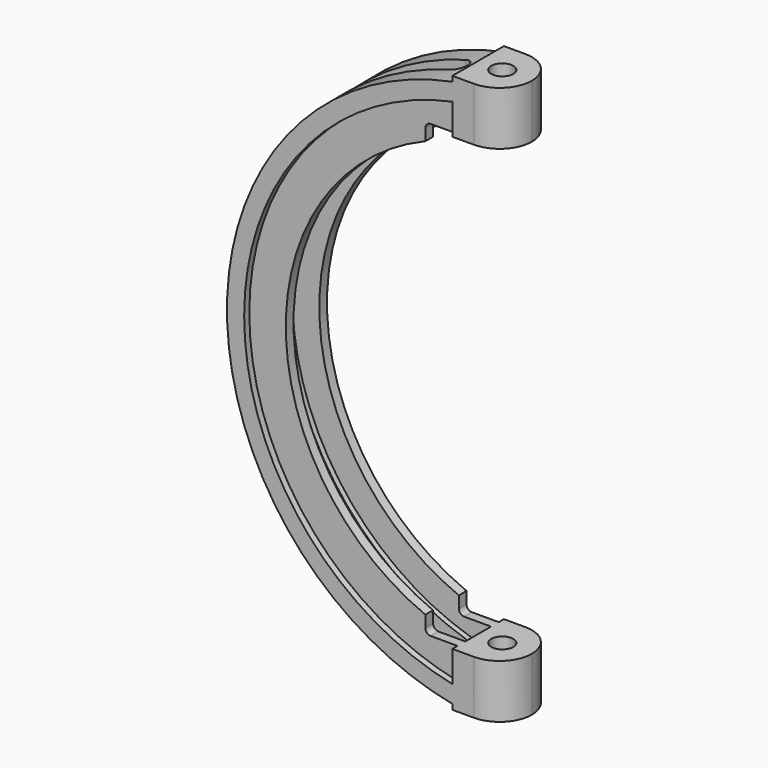
from build123d import *

# Parameters (mm, degrees)
F3_W        = 19.05
F3_H        = 15.875
F4_DEPTH    = 15.875
F6_D        = 6.5278
F8_DEPTH    = 165.101
F9_T1_DEPTH = 63.5
F9_T3_DEPTH = 63.5
F11_DEPTH   = 17.1460001


# Not quite as in the source:
# - a fillet or chamfer that OpenCascade refuses, or shapes differently, is made with other operations: its cross-section is extruded or revolved along the edge and cut away or added


with BuildPart() as f2:
    # F2: sweep along a path in F0
    with BuildLine(Plane.XZ) as f2_path:
        ThreePointArc((0, 76.2), (-76.2, 0), (0, -76.2))
    # F1 (on Right) → F2 (sweep)
    with BuildSketch(Plane.YZ):
        Polygon((9.525, 82.55), (0, 82.55), (-9.525, 82.55), (-9.525, 77.47), (-7.62, 77.47), (-7.62, 66.675), (-4.7625, 66.675), (-4.7625, 74.6125), (0, 74.6125), (4.7625, 74.6125), (4.7625, 66.675), (7.62, 66.675), (7.62, 77.47), (9.525, 77.47), align=None)
    sweep(path=f2_path.line)

    # F3 (on face) → F4 (join)
    with BuildSketch(Plane.YZ):
        with Locations((0, 74.6125)):
            Rectangle(F3_W, F3_H)
        with Locations((0, -74.6125)):
            Rectangle(F3_W, F3_H)
    extrude(amount=-F4_DEPTH)

    # F6 (through all)
    with Locations(Plane.XY.offset(82.55)):
        with Locations((-8.73125, 0)):
            Hole(F6_D / 2)

    # F7 (on face) → F8 (cut, through all)
    with BuildSketch(Plane.XY.offset(82.55)):
        with BuildLine():
            Line((-22.225, 3.175), (-114.3, 3.175))
            Line((-114.3, 3.175), (-114.3, -3.175))
            Line((-114.3, -3.175), (-22.225, -3.175))
            ThreePointArc((-22.225, -3.175), (-19.9799359697, -2.2450640303), (-19.05, 0))
            ThreePointArc((-19.05, 0), (-19.9799359697, 2.2450640303), (-22.225, 3.175))
        make_face()
    extrude(amount=-F8_DEPTH, mode=Mode.SUBTRACT)

    # F9: fillet of radius 9.525 on 4 edges, made by hand

    # F9_s2 → F9_t1 (cut)
    with BuildSketch(Plane.XY.offset(42.8625)):
        with BuildLine():
            ThreePointArc((0, 0), (-2.7898079092, -6.7351920908), (-9.525, -9.525))
            Line((-9.525, -9.525), (0, -9.525))
            Line((0, -9.525), (0, 0))
        make_face()
        with BuildLine():
            ThreePointArc((0, 0), (-2.7898079092, 6.7351920908), (-9.525, 9.525))
            Line((-9.525, 9.525), (0, 9.525))
            Line((0, 9.525), (0, 0))
        make_face()
    extrude(amount=F9_T1_DEPTH, mode=Mode.SUBTRACT)

    # F9_s4 → F9_t3 (cut)
    with BuildSketch(Plane.XY.offset(-106.3625)):
        with BuildLine():
            ThreePointArc((-9.525, -9.525), (-2.7898079092, -6.7351920908), (0, 0))
            Line((0, 0), (0, -9.525))
            Line((0, -9.525), (-9.525, -9.525))
        make_face()
        with BuildLine():
            ThreePointArc((-9.525, 9.525), (-2.7898079092, 6.7351920908), (0, 0))
            Line((0, 0), (0, 9.525))
            Line((0, 9.525), (-9.525, 9.525))
        make_face()
    extrude(amount=F9_T3_DEPTH, mode=Mode.SUBTRACT)

    # F10 (on face) → F11 (cut, through all)
    with BuildSketch(Plane.XZ.offset(7.62)):
        with BuildLine():
            Line((0, 60.325), (0, 66.675))
            Line((0, 66.675), (-23.8125, 66.675))
            ThreePointArc((-23.8125, 66.675), (-24.9350320151, 66.2100320151), (-25.4, 65.0875))
            Line((-25.4, 65.0875), (-25.4, 60.325))
            Line((-25.4, 60.325), (0, 60.325))
        make_face()
        with BuildLine():
            Line((-23.8125, -66.675), (0, -66.675))
            Line((0, -66.675), (0, -60.325))
            Line((0, -60.325), (-25.4, -60.325))
            Line((-25.4, -60.325), (-25.4, -65.0875))
            ThreePointArc((-25.4, -65.0875), (-24.9350320151, -66.2100320151), (-23.8125, -66.675))
        make_face()
    extrude(amount=-F11_DEPTH, mode=Mode.SUBTRACT)


solid = f2.part
